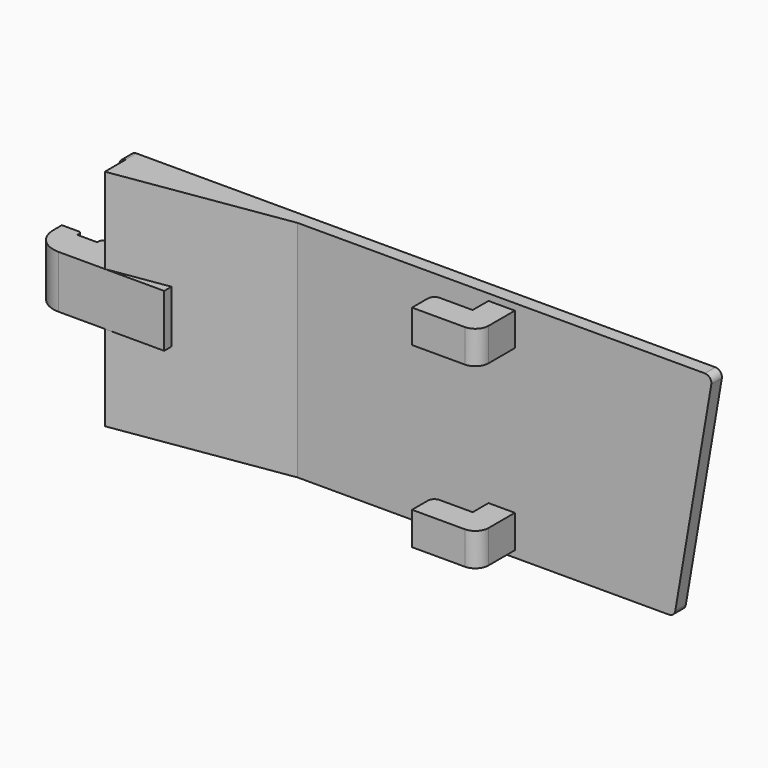
from build123d import *

# Parameters (mm, degrees)
F0_W      = 14
F0_H      = 11
F1_DEPTH  = 0.5
F3_START  = -0.6
F2_W      = 1.5
F2_H      = 4
F2_W_2    = 2
F2_W_3    = 5
F3_DEPTH  = 2.4
F5_START  = -0.2
F5_DEPTH  = 0.4
F6_DEPTH  = 8
F7_R      = 0.5
F8_R      = 1
F9_R      = 0.5
F10_R     = 2
F11_R     = 0.25
F12_START = 0.5
F12_DEPTH = 3.5
F14_DEPTH = 8.5


# Not quite as in the source:
# - a feature names something its author has since deleted; it is built from what else it names


with BuildPart() as f1:
    # F0 (on Front) → F1 (new body, symmetric)
    with BuildSketch(Plane.XZ):
        Polygon((-21.05, -8.5), (21.05, -8.5), (23.95, 8.5), (-21.05, 8.5), align=None)
        with Locations((7.95, 0)):
            Rectangle(F0_W, F0_H, mode=Mode.SUBTRACT)
        with Locations((7.95, 0)):
            Rectangle(F0_W, F0_H)
    extrude(amount=F1_DEPTH, both=True)

    # F2 (on face) → F3 (join)
    with BuildSketch(Plane(origin=(0, 0.5, 0), x_dir=(-1, 0, 0), z_dir=(0, 1, 0)).offset(F3_START)):
        with Locations((25.3, 0)):
            Rectangle(F2_W, F2_H)
        with Locations((22.05, 0)):
            Rectangle(F2_W_2, F2_H)
        with Locations((23.8, 0)):
            Rectangle(F2_W, F2_H)
        with Locations((18.55, 0)):
            Rectangle(F2_W_3, F2_H)
    extrude(amount=-F3_DEPTH)

    # F2 (on face) → F5 (join)
    with BuildSketch(Plane(origin=(0, 0.5, 0), x_dir=(-1, 0, 0), z_dir=(0, 1, 0)).offset(F5_START)):
        with Locations((25.3, 0)):
            Rectangle(F2_W, F2_H)
        with Locations((22.05, 0)):
            Rectangle(F2_W_2, F2_H)
    extrude(amount=-F5_DEPTH)

    # F4 (on Top) → F6 (join, symmetric)
    with BuildSketch(Plane.XY):
        Polygon((3.95, -4), (8.95, -4), (8.95, -0.5), (6.95, -0.5), (6.95, -2), (3.95, -2), align=None)
    extrude(amount=F6_DEPTH, both=True)

    # F7
    f7_edges = [f1.edges().sort_by_distance(p)[0] for p in [
        (-21.05, 0, 8.5),
        (-21.05, 0, -8.5),
        (23.95, 0, 8.5),
        (21.05, 0, -8.5),
    ]]
    fillet(f7_edges, radius=F7_R)

    # F8
    f8_edges = [f1.edges().sort_by_distance(p)[0] for p in [
        (8.95, -4, 0),
    ]]
    fillet(f8_edges, radius=F8_R)

    # F9
    f9_edges = [f1.edges().sort_by_distance(p)[0] for p in [
        (3.95, -2, 0),
    ]]
    fillet(f9_edges, radius=F9_R)

    # F10
    f10_edges = [f1.edges().sort_by_distance(p)[0] for p in [
        (-26.05, -2.5, 0),
    ]]
    fillet(f10_edges, radius=F10_R)

    # F11
    f11_edges = [f1.edges().sort_by_distance(p)[0] for p in [
        (-24.55, 0.3, 0),
        (-23.05, 0.3, 0),
    ]]
    fillet(f11_edges, radius=F11_R)

    # F0 (on Front) → F12 (cut)
    with BuildSketch(Plane.XZ.offset(F12_START)):
        with Locations((7.95, 0)):
            Rectangle(F0_W, F0_H)
    extrude(amount=F12_DEPTH, mode=Mode.SUBTRACT)

    # F13 (on Top) → F14 (join, symmetric)
    with BuildSketch(Plane.XY):
        Polygon((-4.276, 0), (-20.55, 0), (-20.55, -2.5), align=None)
    extrude(amount=F14_DEPTH, both=True)


solid = f1.part
